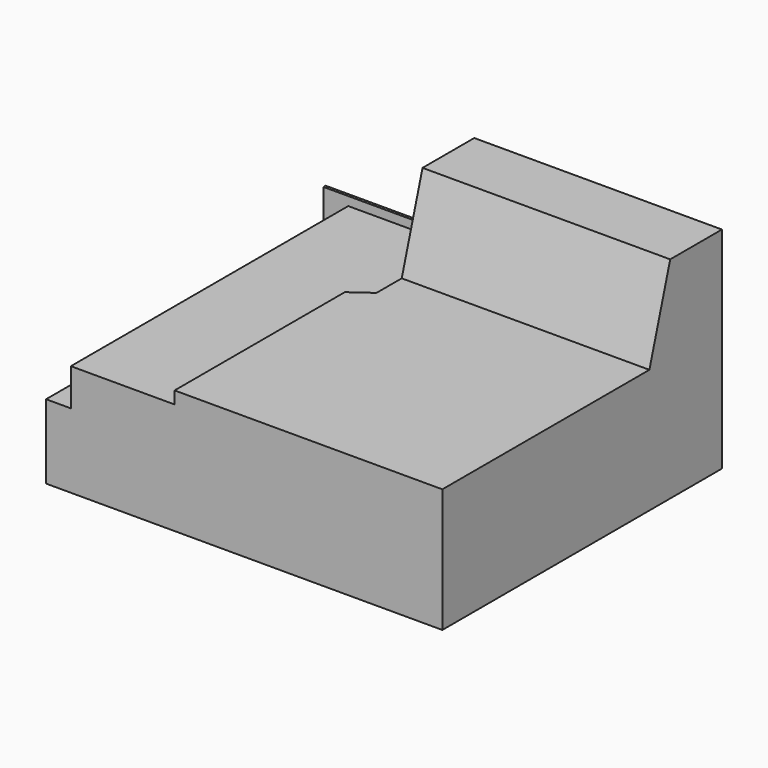
from build123d import *

# Parameters (mm, degrees)
F0_W        = 16
F0_H        = 14
F1_DEPTH    = 5
F2_W        = 1
F2_H        = 14
F3_DEPTH    = 2
F5_DEPTH    = 0.5
F6_W        = 10
F6_H        = 4
F7_DEPTH    = 3.5
F8_T4_DEPTH = 35.959416678
F10_DEPTH   = 0.11
F11_R       = 0.3
F12_DEPTH   = 2.3


# Not quite as in the source:
# - a fillet or chamfer that OpenCascade refuses, or shapes differently, is made with other operations: its cross-section is extruded or revolved along the edge and cut away or added


with BuildPart() as f1:
    # F0 (on Top) → F1 (new body)
    with BuildSketch(Plane.XY):
        with Locations((-8, 7)):
            Rectangle(F0_W, F0_H)
    extrude(amount=F1_DEPTH)

    # F2 (on face) → F3 (cut)
    with BuildSketch(Plane.XY.offset(5)):
        with Locations((-15.5, 7)):
            Rectangle(F2_W, F2_H)
    extrude(amount=-F3_DEPTH, mode=Mode.SUBTRACT)

    # F4 (on face) → F5 (cut, symmetric)
    with BuildSketch(Plane.XY.offset(5)):
        Polygon((-10, 14), (-15, 14), (-15, 0), (-10.8115321142, 0), (-10.8115321142, 8.5921764899), (-10, 9.1764843091), align=None)
    extrude(amount=F5_DEPTH, both=True, mode=Mode.SUBTRACT)

    # F6 (on face) → F7 (join)
    with BuildSketch(Plane.XY.offset(5)):
        with Locations((-5, 12)):
            Rectangle(F6_W, F6_H)
    extrude(amount=F7_DEPTH)

    # F8: chamfer of 5 x 1.5 on 1 edges, made by hand


with BuildPart() as f8_tool2:
    # F8_s3 → F8_t4 (new body)
    with BuildSketch(Plane.YZ.offset(-22.979708339)):
        Polygon((10, 3.5), (11.5, 8.5), (10, 8.5), align=None)
    extrude(amount=F8_T4_DEPTH)

    split(bisect_by=Plane.XY.offset(5), keep=Keep.TOP)


with BuildPart() as f1_1:
    add(f1.part)

    # F8_t1: cut F8_tool2
    add(f8_tool2.part, mode=Mode.SUBTRACT)

    # F9 (on face) → F10 (join)
    with BuildSketch(Plane(origin=(0, 14, 0), x_dir=(-1, 0, 0), z_dir=(0, 1, 0))):
        Polygon((15, 4.8544388264), (10, 4.8544388264), (10, 0), (16, 0), (16, 3), (16, 4.8544388264), align=None)
        Polygon((10, 4.5), (10, 4.8544388264), (10, 8.5), (0, 8.5), (0, 0), (10, 0), align=None)
    extrude(amount=F10_DEPTH)

    # F11 (on face) → F12 (cut)
    with BuildSketch(Plane(origin=(0, 14.11, 0), x_dir=(-1, 0, 0), z_dir=(0, 1, 0))):
        with Locations((1.9506971954, 7.1659904264)):
            Circle(F11_R)
        with Locations((2.8280317048, 7.026860631)):
            Circle(F11_R)
        with Locations((4.8750384645, 7.7731783739)):
            Circle(F11_R)
        with Locations((3.1497415967, 6.2874185075)):
            Circle(F11_R)
        with Locations((2.0762382736, 6.2197762835)):
            Circle(F11_R)
        with BuildLine():
            ThreePointArc((0.9178482584, 2.5111044793), (0.6178482584, 2.8111044793), (0.3178482584, 2.5111044793))
            ThreePointArc((0.3178482584, 2.5111044793), (0.6178482584, 2.2111044793), (0.9178482584, 2.5111044793))
        make_face()
        with Locations((1.2844419159, 2.2510312947)):
            Circle(F11_R)
        with Locations((2.223139369, 2.0780317048)):
            Circle(F11_R)
        with Locations((1.6878734876, 3.0424325256)):
            Circle(F11_R)
        with Locations((2.2534648226, 4.0737193912)):
            Circle(F11_R)
        with Locations((2.3235260528, 4.8911064992)):
            Circle(F11_R)
        with Locations((2.6314037386, 5.6515284814)):
            Circle(F11_R)
        with Locations((1.4768216261, 4.1250384645)):
            Circle(F11_R)
        with BuildLine():
            ThreePointArc((0.9178482584, 4.0984628722), (0.6178482584, 4.3984628722), (0.3178482584, 4.0984628722))
            ThreePointArc((0.3178482584, 4.0984628722), (0.6178482584, 3.7984628722), (0.9178482584, 4.0984628722))
        make_face()
        with Locations((0.8485789713, 3.4970383785)):
            Circle(F11_R)
        with Locations((0.8190860416, 4.816750592)):
            Circle(F11_R)
        with BuildLine():
            ThreePointArc((0.9178482584, 5.5358964019), (0.6178482584, 5.8358964019), (0.3178482584, 5.5358964019))
            ThreePointArc((0.3178482584, 5.5358964019), (0.6178482584, 5.2358964019), (0.9178482584, 5.5358964019))
        make_face()
        with Locations((1.1988501004, 6.0809853088)):
            Circle(F11_R)
        with BuildLine():
            ThreePointArc((2.736303091, 8.1066926941), (3.0010312947, 7.6655580841), (3.2657594984, 8.1066926941))
            Line((3.2657594984, 8.1066926941), (2.736303091, 8.1066926941))
        make_face()
        with BuildLine():
            ThreePointArc((2.3086588338, 7.8268786892), (2.2561014313, 7.9965022753), (2.1168444274, 8.1066926941))
            Line((2.1168444274, 8.1066926941), (1.9004732402, 8.1066926941))
            ThreePointArc((1.9004732402, 8.1066926941), (1.8390352477, 7.5794360918), (2.3086588338, 7.8268786892))
        make_face()
        with Locations((3.7924325256, 7.5621265124)):
            Circle(F11_R)
        with Locations((4.6189634766, 6.9756818416)):
            Circle(F11_R)
        with Locations((3.3696561493, 5.288646793)):
            Circle(F11_R)
        with Locations((3.1127397891, 4.6683982895)):
            Circle(F11_R)
        with Locations((3.8232160392, 5.7836191645)):
            Circle(F11_R)
        with Locations((3.0834548634, 3.9976847774)):
            Circle(F11_R)
        with Locations((3.2853335664, 3.3574042049)):
            Circle(F11_R)
        with Locations((2.8300085443, 2.5571717702)):
            Circle(F11_R)
        with Locations((3.4253850562, 1.9927631688)):
            Circle(F11_R)
        with Locations((2.0840095736, 1.2006971954)):
            Circle(F11_R)
        with Locations((3.0302237165, 1.3262382736)):
            Circle(F11_R)
        with BuildLine():
            ThreePointArc((3.4639975022, 0.5034865462), (3.1690146912, 0.7488501004), (2.8740318802, 0.5034865462))
            Line((2.8740318802, 0.5034865462), (3.4639975022, 0.5034865462))
        make_face()
        with Locations((4.0301234909, 0.8606430113)):
            Circle(F11_R)
        with Locations((4.2602388243, 2.4640656129)):
            Circle(F11_R)
        with Locations((4.9156774171, 2.3187574119)):
            Circle(F11_R)
        with Locations((6.1767839608, 2.7163808355)):
            Circle(F11_R)
        with Locations((6.6303438507, 3.211353207)):
            Circle(F11_R)
        with Locations((6.8872602109, 3.8316017105)):
            Circle(F11_R)
        with Locations((6.9165451366, 4.5023152226)):
            Circle(F11_R)
        with Locations((6.7146664336, 5.1425957951)):
            Circle(F11_R)
        with Locations((5.7397611757, 6.0359343871)):
            Circle(F11_R)
        with Locations((5.0843225829, 6.1812425881)):
            Circle(F11_R)
        with Locations((4.4187134422, 6.0936144309)):
            Circle(F11_R)
        with Locations((6.9697762835, 7.1737617264)):
            Circle(F11_R)
        with Locations((6.2206041032, 6.7167095404)):
            Circle(F11_R)
        with Locations((7.9159904264, 7.2993028046)):
            Circle(F11_R)
        with Locations((8.6122723296, 6.9872750901)):
            Circle(F11_R)
        with Locations((7.776860631, 6.4219682952)):
            Circle(F11_R)
        with Locations((6.8934514885, 6.2473411813)):
            Circle(F11_R)
        with Locations((7.3980573997, 5.600500293)):
            Circle(F11_R)
        with Locations((8.7155580841, 6.2489687053)):
            Circle(F11_R)
        with Locations((9.0350275859, 5.6900447235)):
            Circle(F11_R)
        with Locations((8.3121265124, 5.4575674744)):
            Circle(F11_R)
        with Locations((7.6895853873, 4.8336615271)):
            Circle(F11_R)
        with BuildLine():
            Line((9.4149392098, 4.8595804226), (9.4149392098, 5.1463428204))
            ThreePointArc((9.4149392098, 5.1463428204), (8.8514210287, 5.0029616215), (9.4149392098, 4.8595804226))
        make_face()
        with Locations((7.7421319101, 4.0149618731)):
            Circle(F11_R)
        with Locations((7.5510279791, 3.2171463882)):
            Circle(F11_R)
        with Locations((7.9237617264, 2.2802237165)):
            Circle(F11_R)
        with Locations((7.1332540171, 2.5111044793)):
            Circle(F11_R)
        with Locations((8.8011498996, 2.4190146912)):
            Circle(F11_R)
        with Locations((8.6861317977, 1.6665054718)):
            Circle(F11_R)
        with Locations((8.0493028046, 1.3340095736)):
            Circle(F11_R)
        with Locations((7.1719682952, 1.473139369)):
            Circle(F11_R)
        with Locations((5.7830224588, 1.6115523195)):
            Circle(F11_R)
        with Locations((4.9705388617, 1.4979712257)):
            Circle(F11_R)
        with BuildLine():
            Line((4.9246581604, 0.5034865462), (5.3252649106, 0.5034865462))
            ThreePointArc((5.3252649106, 0.5034865462), (5.1249615355, 1.0268216261), (4.9246581604, 0.5034865462))
        make_face()
        with BuildLine():
            Line((6.7005700373, 0.5034865462), (7.2973673733, 0.5034865462))
            ThreePointArc((7.2973673733, 0.5034865462), (6.9989687053, 0.8344419159), (6.7005700373, 0.5034865462))
        make_face()
        with Locations((6.2075674744, 0.9378734876)):
            Circle(F11_R)
        with Locations((6.5259310741, 1.9595710684)):
            Circle(F11_R)
        with Locations((5.5812865578, 2.4063855691)):
            Circle(F11_R)
        with Locations((4.160673016, 1.6289199655)):
            Circle(F11_R)
        with Locations((9.0539995581, 3.0424325256)):
            Circle(F11_R)
        with Locations((8.3893569887, 3.2801234909)):
            Circle(F11_R)
        with BuildLine():
            Line((9.4149392098, 3.4955470327), (9.4149392098, 3.8709517832))
            ThreePointArc((9.4149392098, 3.8709517832), (8.8809139584, 3.683249408), (9.4149392098, 3.4955470327))
        make_face()
        with Locations((8.5231783739, 4.3749615355)):
            Circle(F11_R)
        with Locations((3.694026347, 2.8247838586)):
            Circle(F11_R)
        with Locations((1.1956938542, 1.4342324575)):
            Circle(F11_R)
        with Locations((2.427445296, 3.2719955888)):
            Circle(F11_R)
        with Locations((1.6106430113, 5.2198765091)):
            Circle(F11_R)
        with Locations((1.1407076381, 6.8986527622)):
            Circle(F11_R)
        with Locations((3.8324830337, 6.7422749581)):
            Circle(F11_R)
        with Locations((5.4393006869, 6.9668999319)):
            Circle(F11_R)
        with Locations((5.9698765091, 7.6393569887)):
            Circle(F11_R)
    extrude(amount=-F12_DEPTH, mode=Mode.SUBTRACT)


solid = f1_1.part
